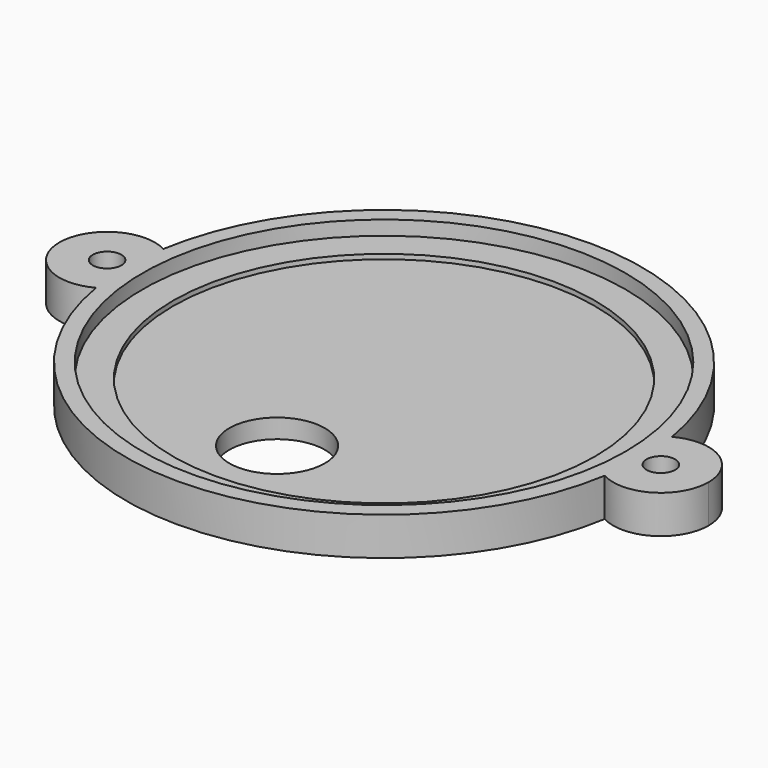
from build123d import *

# Parameters (mm, degrees)
F0_R     = 1.5
F1_DEPTH = 4
F2_DEPTH = 2
F3_R     = 27
F3_R_2   = 22.1
F4_DEPTH = 0.5
F5_R     = 25.3
F6_DEPTH = 1.5
F7_R     = 5
F8_DEPTH = 25


with BuildPart() as f1:
    # F0 (on Top) → F1 (new body)
    with BuildSketch(Plane.XY):
        with BuildLine():
            ThreePointArc((-26.6379310345, -4.4068844099), (-27, 0), (-26.6379310345, 4.4068844099))
            ThreePointArc((-26.6379310345, 4.4068844099), (-34, 0), (-26.6379310345, -4.4068844099))
        make_face()
        with Locations((-29, 0)):
            Circle(F0_R, mode=Mode.SUBTRACT)
    extrude(amount=F1_DEPTH)



with BuildPart() as f1b:
    # F0 (on Top) → F1, piece 2 (new body)
    with BuildSketch(Plane.XY):
        with BuildLine():
            ThreePointArc((26.6379310345, 4.4068844099), (26.9093305187, 2.21086658), (27, 0))
            ThreePointArc((27, 0), (26.9093305187, -2.21086658), (26.6379310345, -4.4068844099))
            ThreePointArc((26.6379310345, -4.4068844099), (31.5680396388, -4.2901249881), (34, 0))
            ThreePointArc((34, 0), (31.5680396388, 4.2901249881), (26.6379310345, 4.4068844099))
        make_face()
        with Locations((29, 0)):
            Circle(F0_R, mode=Mode.SUBTRACT)
    extrude(amount=F1_DEPTH)


with BuildPart() as f2:
    # F0 (on Top) → F2 (new body)
    with BuildSketch(Plane.XY):
        with BuildLine():
            ThreePointArc((-24, 0), (-24.7098750119, 2.5680396388), (-26.6379310345, 4.4068844099))
            ThreePointArc((-26.6379310345, 4.4068844099), (-27, 0), (-26.6379310345, -4.4068844099))
            ThreePointArc((-26.6379310345, -4.4068844099), (-24.7098750119, -2.5680396388), (-24, 0))
        make_face()
        with BuildLine():
            ThreePointArc((26.6379310345, -4.4068844099), (26.9093305187, -2.21086658), (27, 0))
            ThreePointArc((27, 0), (26.9093305187, 2.21086658), (26.6379310345, 4.4068844099))
            ThreePointArc((26.6379310345, 4.4068844099), (24, 0), (26.6379310345, -4.4068844099))
        make_face()
        with BuildLine():
            ThreePointArc((26.6379310345, -4.4068844099), (24, 0), (26.6379310345, 4.4068844099))
            ThreePointArc((26.6379310345, 4.4068844099), (0, 27), (-26.6379310345, 4.4068844099))
            ThreePointArc((-26.6379310345, 4.4068844099), (-24.7098750119, 2.5680396388), (-24, 0))
            ThreePointArc((-24, 0), (-24.7098750119, -2.5680396388), (-26.6379310345, -4.4068844099))
            ThreePointArc((-26.6379310345, -4.4068844099), (0, -27), (26.6379310345, -4.4068844099))
        make_face()
    extrude(amount=F2_DEPTH)


with BuildPart() as f1_1:
    add(f1.part)

    add(f1b.part)  # F4 merges F1b

    add(f2.part)  # F4 merges F2
    # F3 (on face) → F4 (join)
    with BuildSketch(Plane.XY.offset(2)):
        Circle(F3_R)
        Circle(F3_R_2, mode=Mode.SUBTRACT)
    extrude(amount=F4_DEPTH)

    # F5 (on face) → F6 (join)
    with BuildSketch(Plane.XY.offset(2.5)):
        with BuildLine():
            ThreePointArc((26.6379310345, -4.4068844099), (27, 0), (26.6379310345, 4.4068844099))
            ThreePointArc((26.6379310345, 4.4068844099), (0, 27), (-26.6379310345, 4.4068844099))
            ThreePointArc((-26.6379310345, 4.4068844099), (-27, 0), (-26.6379310345, -4.4068844099))
            ThreePointArc((-26.6379310345, -4.4068844099), (0, -27), (26.6379310345, -4.4068844099))
        make_face()
        Circle(F5_R, mode=Mode.SUBTRACT)
    extrude(amount=F6_DEPTH)

    # F7 (on face) → F8 (cut)
    with BuildSketch(Plane.XY.offset(2)):
        with Locations((0, -14)):
            Circle(F7_R)
    extrude(amount=-F8_DEPTH, mode=Mode.SUBTRACT)


solid = f1_1.part
